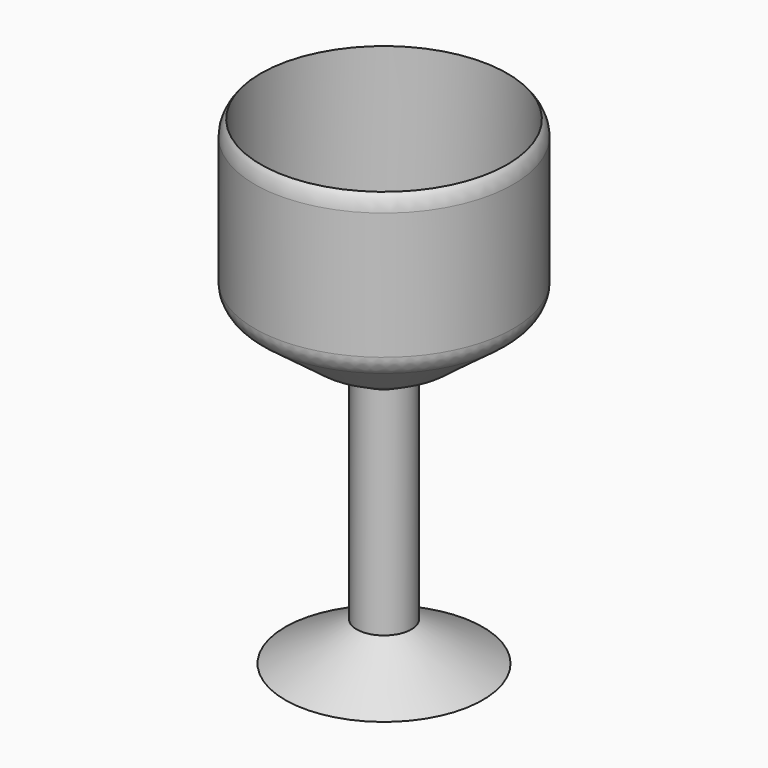
from build123d import *

# Parameters (mm, degrees)
F2_T = -1.27
F4_R = 5.08


# Not quite as in the source:
# - a fillet or chamfer that OpenCascade refuses, or shapes differently, is made with other operations: its cross-section is extruded or revolved along the edge and cut away or added


with BuildPart() as f1:
    # F0 (on Front) → F1 (revolve)
    with BuildSketch(Plane.XZ):
        Polygon((0, -54.0067516267), (0, 47.3392494023), (-27.3367501795, 47.3392494023), (-27.3367501795, 14.6685000509), (-13.1127499044, 4.0005003102), (-5.7784998789, 0), (-5.7784998789, -45.7835011184), (-20.8915006369, -54.0067516267), align=None)
    revolve(axis=Axis((0, 0, -3.3337511122), (0, 0, -1)))

    # F2
    f2_openings = [f1.faces().sort_by_distance(p)[0] for p in [
        (0, 0, 47.339249),
    ]]
    offset(amount=F2_T, openings=f2_openings, kind=Kind.INTERSECTION)

    # F3: fillet of radius 5.08 on 1 edges, made by hand

    # F3_s1 → F3_t2 (revolve, cut)
    with BuildSketch(Plane.XZ):
        with BuildLine():
            ThreePointArc((-27.3371501795, 43.9787802623), (-27.0090313843, 45.775143597), (-26.0670501985, 47.3395139559))
            Line((-26.0670501985, 47.3395139559), (-26.448176769, 47.6755873252))
            ThreePointArc((-26.448176769, 47.6755873252), (-26.701900189, 47.8473859708), (-27.3367501795, 47.8473859708))
            Line((-27.3367501795, 47.8473859708), (-27.8448867481, 47.3392494023))
            ThreePointArc((-27.8448867481, 47.3392494023), (-27.8448867481, 45.6590148323), (-27.8452867481, 43.9787802623))
            Line((-27.8452867481, 43.9787802623), (-27.3371501795, 43.9787802623))
        make_face()
    revolve(axis=Axis((0, 0, 47.3392494023), (0, 0, -1)), mode=Mode.SUBTRACT)

    # F4
    f4_edges = [f1.edges().sort_by_distance(p)[0] for p in [
        (27.33675, 0, 14.6685),
        (13.11275, 0, 4.0005),
        (-20.22475, 0, 9.3345),
    ]]
    fillet(f4_edges, radius=F4_R)


solid = f1.part
